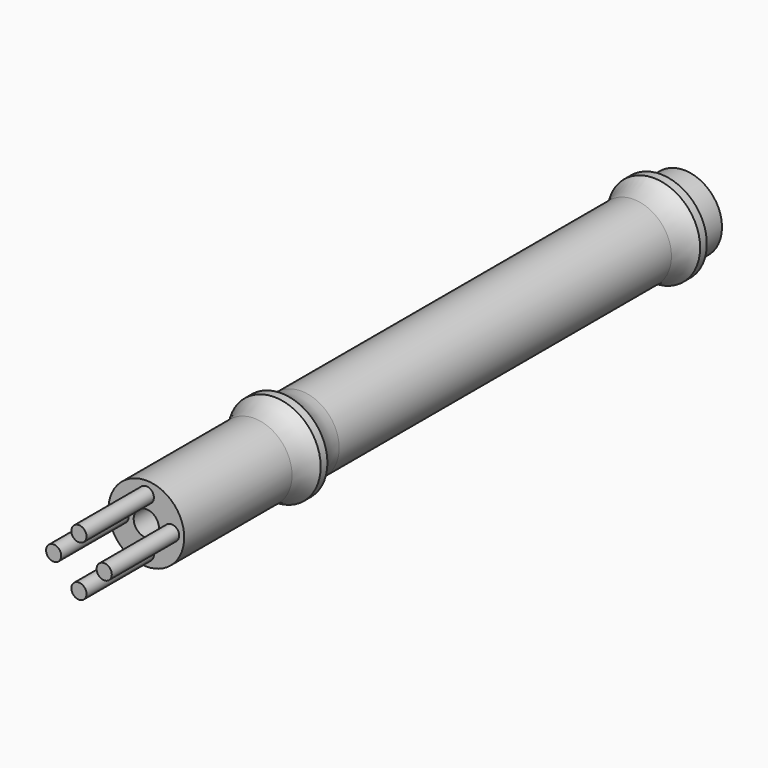
from build123d import *

# Parameters (mm, degrees)
F0_R      = 4.5
F1_DEPTH  = 19
F2_DEPTH  = 57.3
F3_R      = 5.5
F4_DEPTH  = 1
F6_R      = 1.5
F7_DEPTH  = 10
F8_R      = 0.9
F9_DEPTH  = 10
F10_R     = 4.5
F12_DEPTH = 3.5
F11_R     = 5.5
F11_R_2   = 4.5
F13_DEPTH = 1


# Not quite as in the source:
# - a fillet or chamfer that OpenCascade refuses, or shapes differently, is made with other operations: its cross-section is extruded or revolved along the edge and cut away or added


with BuildPart() as f1:
    # F0 (on Front) → F1 (new body)
    with BuildSketch(Plane.XZ):
        Circle(F0_R)
    extrude(amount=F1_DEPTH)

    # F2 (add): a face of the model
    f2_faces = [f1.faces().sort_by_distance(p)[0] for p in [
        (0, 0, 0),
    ]]
    extrude(f2_faces, amount=F2_DEPTH)

    # F3 (on Front) → F4 (join)
    with BuildSketch(Plane.XZ):
        Circle(F3_R)
    extrude(amount=-F4_DEPTH)

    # F5: fillet of radius 5 on 2 edges, made by hand

    # F5_s1 → F5_t2 (revolve)
    with BuildSketch(Plane.XY):
        with BuildLine():
            ThreePointArc((4.5, -3), (4.7565835097, -1.4188611699), (5.5, 0))
            Line((5.5, 0), (4.5, 0))
            Line((4.5, 0), (4.5, -3))
        make_face()
    revolve(axis=Axis((0, 0, 0), (0, -1, 0)))

    # F5_s3 → F5_t4 (revolve)
    with BuildSketch(Plane.XY):
        with BuildLine():
            ThreePointArc((5.5, 1), (4.7565835097, 2.4188611699), (4.5, 4))
            Line((4.5, 4), (4.5, 1))
            Line((4.5, 1), (5.5, 1))
        make_face()
    revolve(axis=Axis((0, 1, 0), (0, -1, 0)))

    # F6 (on face) → F7 (cut)
    with BuildSketch(Plane.XZ.offset(19)):
        Circle(F6_R)
    extrude(amount=-F7_DEPTH, mode=Mode.SUBTRACT)

    # F8 (on face) → F9 (join)
    with BuildSketch(Plane.XZ.offset(19)):
        with Locations((-3, 0)):
            Circle(F8_R)
        with Locations((0, -3)):
            Circle(F8_R)
        with Locations((3, 0)):
            Circle(F8_R)
        with Locations((0, 3)):
            Circle(F8_R)
    extrude(amount=F9_DEPTH)

    # F10 (on face) → F12 (join)
    with BuildSketch(Plane(origin=(0, 57.3, 0), x_dir=(-1, 0, 0), z_dir=(0, 1, 0))):
        Circle(F10_R)
    extrude(amount=F12_DEPTH)

    # F11 (on face) → F13 (join)
    with BuildSketch(Plane(origin=(0, 57.3, 0), x_dir=(-1, 0, 0), z_dir=(0, 1, 0))):
        Circle(F11_R)
        Circle(F11_R_2, mode=Mode.SUBTRACT)
    extrude(amount=-F13_DEPTH)

    # F14: fillet of radius 5 on 1 edges, made by hand

    # F14_s1 → F14_t2 (revolve)
    with BuildSketch(Plane.XY):
        with BuildLine():
            ThreePointArc((4.5, 53.3), (4.7565835097, 54.8811388301), (5.5, 56.3))
            Line((5.5, 56.3), (4.5, 56.3))
            Line((4.5, 56.3), (4.5, 53.3))
        make_face()
    revolve(axis=Axis((0, 56.3, 0), (0, -1, 0)))


solid = f1.part
